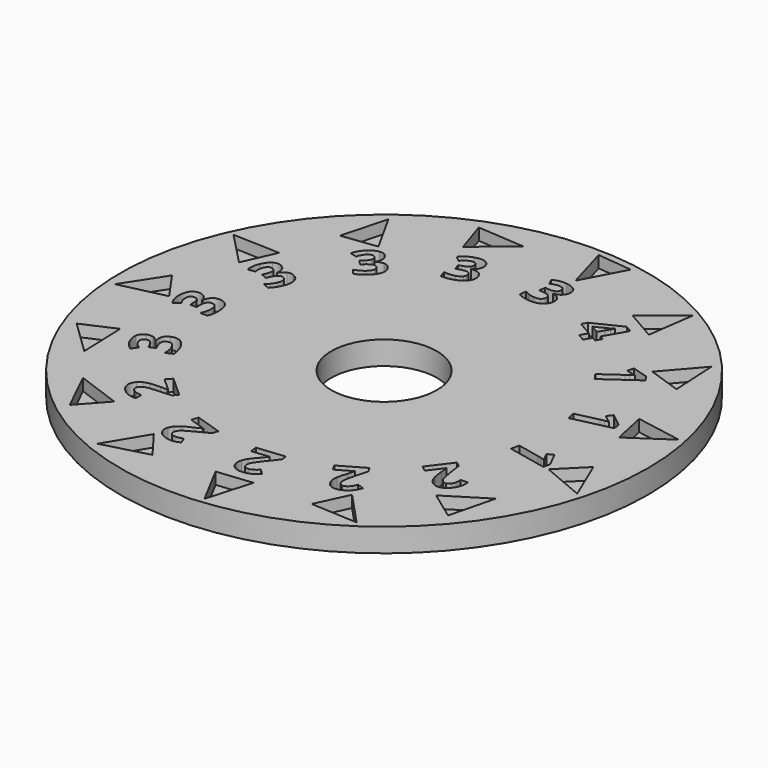
from build123d import *

# Parameters (mm, degrees)
F1_R           = 22.5
F1_R_2         = 4.5
F2_DEPTH       = 2
F1_TEXT_SIZE   = 4.7496985644
F1_TEXT_SIZE_2 = 4.7488933279
F3_DEPTH       = 1


# Not quite as in the source:
# - Text() gives the source's letters only with a copy of the font that has no kerning and outlines rounded to 1/6400 em; it was checked with that copy


with BuildPart() as f2:
    # F1 (on Top) → F2 (new body)
    with BuildSketch(Plane.XY):
        Circle(F1_R)
        Polygon((-11.2424762449, -14.7004235416), (-13.249868064, -16.929858018), (-15.0018269196, -13.3339380845), align=None, mode=Mode.SUBTRACT)
        Polygon((-6.25651676, -16.7168305622), (-4.4510716905, -19.1127370923), (-8.3152139559, -20.1463736594), align=None, mode=Mode.SUBTRACT)
        with BuildLine():
            Line((-10.6299594554, -10.1070689959), (-10.2262327152, -9.6586850257))
            Line((-10.2262327152, -9.6586850257), (-8.4646848666, -11.2447898327))
            Line((-8.4646848666, -11.2447898327), (-8.7983925781, -11.6154097934))
            Line((-8.7983925781, -11.6154097934), (-10.0065299775, -11.6850315037))
            add(Edge.make_bspline(
                [(-10.0065299775, -11.6850315037), (-10.5470234377, -11.7196634778), (-10.7331228689, -11.7533264526)],
                knots=[0, 0, 0, 1, 1, 1], degree=2))
            add(Edge.make_bspline(
                [(-10.7331228689, -11.7533264526), (-10.9192223, -11.7869894275), (-11.0426903114, -11.8475858577)],
                knots=[0, 0, 0, 1, 1, 1], degree=2))
            add(Edge.make_bspline(
                [(-11.0426903114, -11.8475858577), (-11.1661583227, -11.908182288), (-11.2575306723, -12.0096615629)],
                knots=[0, 0, 0, 1, 1, 1], degree=2))
            add(Edge.make_bspline(
                [(-11.2575306723, -12.0096615629), (-11.3940926078, -12.1613289575), (-11.3770531036, -12.3109896076)],
                knots=[0, 0, 0, 1, 1, 1], degree=2))
            add(Edge.make_bspline(
                [(-11.3770531036, -12.3109896076), (-11.3600135994, -12.4606502577), (-11.2204795964, -12.5862872383)],
                knots=[0, 0, 0, 1, 1, 1], degree=2))
            add(Edge.make_bspline(
                [(-11.2204795964, -12.5862872383), (-11.0743273797, -12.7178832852), (-10.8758640896, -12.7747453279)],
                knots=[0, 0, 0, 1, 1, 1], degree=2))
            add(Edge.make_bspline(
                [(-10.8758640896, -12.7747453279), (-10.6774007995, -12.8316073705), (-10.4156554656, -12.8425880348)],
                knots=[0, 0, 0, 1, 1, 1], degree=2))
            Line((-10.4156554656, -12.8425880348), (-10.43498689, -13.446341255))
            add(Edge.make_bspline(
                [(-10.43498689, -13.446341255), (-10.7638659788, -13.4378279364), (-10.9451487095, -13.3929400695)],
                knots=[0, 0, 0, 1, 1, 1], degree=2))
            add(Edge.make_bspline(
                [(-10.9451487095, -13.3929400695), (-11.1264314403, -13.3480522025), (-11.3029865492, -13.2529947668)],
                knots=[0, 0, 0, 1, 1, 1], degree=2))
            add(Edge.make_bspline(
                [(-11.3029865492, -13.2529947668), (-11.4795416581, -13.1579373311), (-11.6587849426, -12.9965459528)],
                knots=[0, 0, 0, 1, 1, 1], degree=2))
            add(Edge.make_bspline(
                [(-11.6587849426, -12.9965459528), (-11.8948345604, -12.7840059223), (-11.9982645368, -12.5350880009)],
                knots=[0, 0, 0, 1, 1, 1], degree=2))
            add(Edge.make_bspline(
                [(-11.9982645368, -12.5350880009), (-12.1016945131, -12.2861700794), (-12.0620052305, -12.0407869417)],
                knots=[0, 0, 0, 1, 1, 1], degree=2))
            add(Edge.make_bspline(
                [(-12.0620052305, -12.0407869417), (-12.0223159479, -11.795403804), (-11.8425507819, -11.5957543609)],
                knots=[0, 0, 0, 1, 1, 1], degree=2))
            add(Edge.make_bspline(
                [(-11.8425507819, -11.5957543609), (-11.6856287033, -11.4214747366), (-11.4871034089, -11.3241014284)],
                knots=[0, 0, 0, 1, 1, 1], degree=2))
            add(Edge.make_bspline(
                [(-11.4871034089, -11.3241014284), (-11.2885781145, -11.2267281201), (-11.0158154046, -11.1822174032)],
                knots=[0, 0, 0, 1, 1, 1], degree=2))
            add(Edge.make_bspline(
                [(-11.0158154046, -11.1822174032), (-10.7430526948, -11.1377066862), (-10.1521469424, -11.1324877692)],
                knots=[0, 0, 0, 1, 1, 1], degree=2))
            Line((-10.1521469424, -11.1324877692), (-9.5532408393, -11.1194926742))
            Line((-9.5532408393, -11.1194926742), (-9.5318875185, -11.0957774088))
            Line((-9.5318875185, -11.0957774088), (-10.6299594554, -10.1070689959))
        make_face(mode=Mode.SUBTRACT)
        with BuildLine():
            Line((-5.6002424488, -13.5567744278), (-5.41379391, -12.9829448295))
            Line((-5.41379391, -12.9829448295), (-3.1594129297, -13.7154376128))
            Line((-3.1594129297, -13.7154376128), (-3.313525375, -14.1897469487))
            Line((-3.313525375, -14.1897469487), (-4.3888961077, -14.7447432961))
            add(Edge.make_bspline(
                [(-4.3888961077, -14.7447432961), (-4.8685753604, -14.9962196744), (-5.0248936849, -15.10266579)],
                knots=[0, 0, 0, 1, 1, 1], degree=2))
            add(Edge.make_bspline(
                [(-5.0248936849, -15.10266579), (-5.1812120095, -15.2091119056), (-5.2693588619, -15.3146884637)],
                knots=[0, 0, 0, 1, 1, 1], degree=2))
            add(Edge.make_bspline(
                [(-5.2693588619, -15.3146884637), (-5.3575057142, -15.4202650218), (-5.3997031695, -15.5501354352)],
                knots=[0, 0, 0, 1, 1, 1], degree=2))
            add(Edge.make_bspline(
                [(-5.3997031695, -15.5501354352), (-5.4627700184, -15.7442352378), (-5.3863311863, -15.8740264542)],
                knots=[0, 0, 0, 1, 1, 1], degree=2))
            add(Edge.make_bspline(
                [(-5.3863311863, -15.8740264542), (-5.3098923542, -16.0038176705), (-5.1313205358, -16.0618391715)],
                knots=[0, 0, 0, 1, 1, 1], degree=2))
            add(Edge.make_bspline(
                [(-5.1313205358, -16.0618391715), (-4.9442789078, -16.1226126804), (-4.7398457943, -16.0938364488)],
                knots=[0, 0, 0, 1, 1, 1], degree=2))
            add(Edge.make_bspline(
                [(-4.7398457943, -16.0938364488), (-4.5354126808, -16.0650602172), (-4.2918301814, -15.9686301347)],
                knots=[0, 0, 0, 1, 1, 1], degree=2))
            Line((-4.2918301814, -15.9686301347), (-4.0639217583, -16.5280489453))
            add(Edge.make_bspline(
                [(-4.0639217583, -16.5280489453), (-4.3678304346, -16.6540388183), (-4.5516979901, -16.6867660406)],
                knots=[0, 0, 0, 1, 1, 1], degree=2))
            add(Edge.make_bspline(
                [(-4.5516979901, -16.6867660406), (-4.7355655457, -16.719493263), (-4.9355200058, -16.7044654068)],
                knots=[0, 0, 0, 1, 1, 1], degree=2))
            add(Edge.make_bspline(
                [(-4.9355200058, -16.7044654068), (-5.1354744658, -16.6894375505), (-5.3648651416, -16.6149040018)],
                knots=[0, 0, 0, 1, 1, 1], degree=2))
            add(Edge.make_bspline(
                [(-5.3648651416, -16.6149040018), (-5.6669550163, -16.5167490515), (-5.8626870411, -16.3314199764)],
                knots=[0, 0, 0, 1, 1, 1], degree=2))
            add(Edge.make_bspline(
                [(-5.8626870411, -16.3314199764), (-6.058419066, -16.1460909013), (-6.1219674158, -15.9057791649)],
                knots=[0, 0, 0, 1, 1, 1], degree=2))
            add(Edge.make_bspline(
                [(-6.1219674158, -15.9057791649), (-6.1855157657, -15.6654674285), (-6.1024968591, -15.4099615065)],
                knots=[0, 0, 0, 1, 1, 1], degree=2))
            add(Edge.make_bspline(
                [(-6.1024968591, -15.4099615065), (-6.0300273163, -15.1869231878), (-5.8882707279, -15.0172207326)],
                knots=[0, 0, 0, 1, 1, 1], degree=2))
            add(Edge.make_bspline(
                [(-5.8882707279, -15.0172207326), (-5.7465141395, -14.8475182773), (-5.5154371445, -14.6959131251)],
                knots=[0, 0, 0, 1, 1, 1], degree=2))
            add(Edge.make_bspline(
                [(-5.5154371445, -14.6959131251), (-5.2843601496, -14.5443079728), (-4.7466636083, -14.2991972328)],
                knots=[0, 0, 0, 1, 1, 1], degree=2))
            Line((-4.7466636083, -14.2991972328), (-4.2048212396, -14.0437285648))
            Line((-4.2048212396, -14.0437285648), (-4.1949598778, -14.0133784139))
            Line((-4.1949598778, -14.0133784139), (-5.6002424488, -13.5567744278))
        make_face(mode=Mode.SUBTRACT)
        Polygon((-20.2206789231, -7.4874351718), (-17.4800425502, -6.2672252426), (-17.3421408981, -10.2648474276), align=None, mode=Mode.SUBTRACT)
        with BuildLine():
            add(Edge.make_bspline(
                [(-16.0555084734, -6.3502361216), (-15.9846522039, -5.9848032435), (-15.63752696, -5.8302531275)],
                knots=[0, 0, 0, 1, 1, 1], degree=2))
            add(Edge.make_bspline(
                [(-15.63752696, -5.8302531275), (-15.3473519515, -5.7010588899), (-15.0656267009, -5.7864377298)],
                knots=[0, 0, 0, 1, 1, 1], degree=2))
            add(Edge.make_bspline(
                [(-15.0656267009, -5.7864377298), (-14.7839014504, -5.8718165696), (-14.5657195033, -6.1556790233)],
                knots=[0, 0, 0, 1, 1, 1], degree=2))
            Line((-14.5657195033, -6.1556790233), (-14.5535158814, -6.1502456208))
            add(Edge.make_bspline(
                [(-14.5535158814, -6.1502456208), (-14.6739633861, -5.7538172162), (-14.5783310232, -5.480524784)],
                knots=[0, 0, 0, 1, 1, 1], degree=2))
            add(Edge.make_bspline(
                [(-14.5783310232, -5.480524784), (-14.4826986603, -5.2072323518), (-14.175574177, -5.0704917219)],
                knots=[0, 0, 0, 1, 1, 1], degree=2))
            add(Edge.make_bspline(
                [(-14.175574177, -5.0704917219), (-13.7287860212, -4.8715688187), (-13.3353417194, -5.0847108089)],
                knots=[0, 0, 0, 1, 1, 1], degree=2))
            add(Edge.make_bspline(
                [(-13.3353417194, -5.0847108089), (-12.9418974175, -5.297852799), (-12.6741514158, -5.8992201649)],
                knots=[0, 0, 0, 1, 1, 1], degree=2))
            add(Edge.make_bspline(
                [(-12.6741514158, -5.8992201649), (-12.4495707785, -6.4036365349), (-12.4434645647, -6.8680328121)],
                knots=[0, 0, 0, 1, 1, 1], degree=2))
            Line((-12.4434645647, -6.8680328121), (-13.0007632961, -7.1161581936))
            add(Edge.make_bspline(
                [(-13.0007632961, -7.1161581936), (-12.9899058705, -6.8960450975), (-13.0289086124, -6.6542629928)],
                knots=[0, 0, 0, 1, 1, 1], degree=2))
            add(Edge.make_bspline(
                [(-13.0289086124, -6.6542629928), (-13.0679113544, -6.4124808881), (-13.1620903313, -6.2009514426)],
                knots=[0, 0, 0, 1, 1, 1], degree=2))
            add(Edge.make_bspline(
                [(-13.1620903313, -6.2009514426), (-13.3066792093, -5.8761995055), (-13.4856738941, -5.7706718458)],
                knots=[0, 0, 0, 1, 1, 1], degree=2))
            add(Edge.make_bspline(
                [(-13.4856738941, -5.7706718458), (-13.6646685788, -5.6651441861), (-13.9087410159, -5.7738122364)],
                knots=[0, 0, 0, 1, 1, 1], degree=2))
            add(Edge.make_bspline(
                [(-13.9087410159, -5.7738122364), (-14.1263722723, -5.8707079146), (-14.1383233267, -6.089276991)],
                knots=[0, 0, 0, 1, 1, 1], degree=2))
            add(Edge.make_bspline(
                [(-14.1383233267, -6.089276991), (-14.1502743812, -6.3078460674), (-13.9767073564, -6.6976839878)],
                knots=[0, 0, 0, 1, 1, 1], degree=2))
            Line((-13.9767073564, -6.6976839878), (-13.8719634301, -6.932942698))
            Line((-13.8719634301, -6.932942698), (-14.3743458632, -7.1566177682))
            Line((-14.3743458632, -7.1566177682), (-14.4809009236, -6.917291184))
            add(Edge.make_bspline(
                [(-14.4809009236, -6.917291184), (-14.6411862978, -6.5572843393), (-14.8095309509, -6.4327984384)],
                knots=[0, 0, 0, 1, 1, 1], degree=2))
            add(Edge.make_bspline(
                [(-14.8095309509, -6.4327984384), (-14.9778756039, -6.3083125375), (-15.2063545242, -6.4100379068)],
                knots=[0, 0, 0, 1, 1, 1], degree=2))
            add(Edge.make_bspline(
                [(-15.2063545242, -6.4100379068), (-15.5582256211, -6.5667010126), (-15.3620194192, -7.0073873574)],
                knots=[0, 0, 0, 1, 1, 1], degree=2))
            add(Edge.make_bspline(
                [(-15.3620194192, -7.0073873574), (-15.2941018877, -7.1599326306), (-15.1729210863, -7.2952625586)],
                knots=[0, 0, 0, 1, 1, 1], degree=2))
            add(Edge.make_bspline(
                [(-15.1729210863, -7.2952625586), (-15.0517402849, -7.4305924866), (-14.8412651329, -7.5675970724)],
                knots=[0, 0, 0, 1, 1, 1], degree=2))
            Line((-14.8412651329, -7.5675970724), (-15.1571916668, -8.0713877192))
            add(Edge.make_bspline(
                [(-15.1571916668, -8.0713877192), (-15.6509420228, -7.7834859121), (-15.9123490549, -7.196356105)],
                knots=[0, 0, 0, 1, 1, 1], degree=2))
            add(Edge.make_bspline(
                [(-15.9123490549, -7.196356105), (-16.1263647428, -6.7156689997), (-16.0555084734, -6.3502361216)],
                knots=[0, 0, 0, 1, 1, 1], degree=2))
        make_face(mode=Mode.SUBTRACT)
        Polygon((0.3273238917, -18.3647082401), (3.3108895778, -18.0511228503), (2.2067086503, -21.8957014331), align=None, mode=Mode.SUBTRACT)
        with BuildLine():
            Line((0.3347819501, -14.5979841554), (0.2717243335, -13.9980310095))
            Line((0.2717243335, -13.9980310095), (2.6287358317, -13.7502991185))
            Line((2.6287358317, -13.7502991185), (2.6808572565, -14.2462013498))
            Line((2.6808572565, -14.2462013498), (1.9243228399, -15.1904483146))
            add(Edge.make_bspline(
                [(1.9243228399, -15.1904483146), (1.5884556461, -15.615214522), (1.4889641565, -15.7760110129)],
                knots=[0, 0, 0, 1, 1, 1], degree=2))
            add(Edge.make_bspline(
                [(1.4889641565, -15.7760110129), (1.389472667, -15.9368075037), (1.3518947371, -16.069086614)],
                knots=[0, 0, 0, 1, 1, 1], degree=2))
            add(Edge.make_bspline(
                [(1.3518947371, -16.069086614), (1.3143168072, -16.2013657243), (1.3285881497, -16.3371484781)],
                knots=[0, 0, 0, 1, 1, 1], degree=2))
            add(Edge.make_bspline(
                [(1.3285881497, -16.3371484781), (1.3499176018, -16.540084659), (1.4725180047, -16.6275495304)],
                knots=[0, 0, 0, 1, 1, 1], degree=2))
            add(Edge.make_bspline(
                [(1.4725180047, -16.6275495304), (1.5951184077, -16.7150144017), (1.7818196942, -16.6953913058)],
                knots=[0, 0, 0, 1, 1, 1], degree=2))
            add(Edge.make_bspline(
                [(1.7818196942, -16.6953913058), (1.9773763777, -16.6748374701), (2.1524012943, -16.5654171897)],
                knots=[0, 0, 0, 1, 1, 1], degree=2))
            add(Edge.make_bspline(
                [(2.1524012943, -16.5654171897), (2.327426211, -16.4559969094), (2.5106971728, -16.2688614487)],
                knots=[0, 0, 0, 1, 1, 1], degree=2))
            Line((2.5106971728, -16.2688614487), (2.9463641336, -16.6871463294))
            add(Edge.make_bspline(
                [(2.9463641336, -16.6871463294), (2.7200128217, -16.9258141311), (2.5653790322, -17.0304798614)],
                knots=[0, 0, 0, 1, 1, 1], degree=2))
            add(Edge.make_bspline(
                [(2.5653790322, -17.0304798614), (2.4107452428, -17.1351455916), (2.2219973789, -17.2027343071)],
                knots=[0, 0, 0, 1, 1, 1], degree=2))
            add(Edge.make_bspline(
                [(2.2219973789, -17.2027343071), (2.033249515, -17.2703230226), (1.7934158466, -17.2955305569)],
                knots=[0, 0, 0, 1, 1, 1], degree=2))
            add(Edge.make_bspline(
                [(1.7934158466, -17.2955305569), (1.477573354, -17.3287269405), (1.2234262199, -17.2390469989)],
                knots=[0, 0, 0, 1, 1, 1], degree=2))
            add(Edge.make_bspline(
                [(1.2234262199, -17.2390469989), (0.9692790858, -17.1493670573), (0.8135076036, -16.9557116414)],
                knots=[0, 0, 0, 1, 1, 1], degree=2))
            add(Edge.make_bspline(
                [(0.8135076036, -16.9557116414), (0.6577361213, -16.7620562255), (0.6296588062, -16.4949184163)],
                knots=[0, 0, 0, 1, 1, 1], degree=2))
            add(Edge.make_bspline(
                [(0.6296588062, -16.4949184163), (0.6051493267, -16.2617262957), (0.6656159542, -16.0490738476)],
                knots=[0, 0, 0, 1, 1, 1], degree=2))
            add(Edge.make_bspline(
                [(0.6656159542, -16.0490738476), (0.7260825818, -15.8364213995), (0.8754932157, -15.6039751344)],
                knots=[0, 0, 0, 1, 1, 1], degree=2))
            add(Edge.make_bspline(
                [(0.8754932157, -15.6039751344), (1.0249038496, -15.3715288692), (1.4163521878, -14.9289832193)],
                knots=[0, 0, 0, 1, 1, 1], degree=2))
            Line((1.4163521878, -14.9289832193), (1.807375051, -14.4752907614))
            Line((1.807375051, -14.4752907614), (1.8040399003, -14.4435589222))
            Line((1.8040399003, -14.4435589222), (0.3347819501, -14.5979841554))
        make_face(mode=Mode.SUBTRACT)
        Polygon((8.2439705729, -18.0201064795), (9.5118253582, -15.3011831184), (12.2385771851, -18.2277552556), align=None, mode=Mode.SUBTRACT)
        with BuildLine():
            Line((6.2546528897, -13.267149647), (5.9529728168, -12.7446244331))
            Line((5.9529728168, -12.7446244331), (8.0057963507, -11.5594262132))
            Line((8.0057963507, -11.5594262132), (8.2551555254, -11.991328973))
            Line((8.2551555254, -11.991328973), (7.9480347187, -13.161850211))
            add(Edge.make_bspline(
                [(7.9480347187, -13.161850211), (7.8139500188, -13.6865919069), (7.7884575235, -13.8739854149)],
                knots=[0, 0, 0, 1, 1, 1], degree=2))
            add(Edge.make_bspline(
                [(7.7884575235, -13.8739854149), (7.7629650282, -14.0613789228), (7.7824419443, -14.1975293063)],
                knots=[0, 0, 0, 1, 1, 1], degree=2))
            add(Edge.make_bspline(
                [(7.7824419443, -14.1975293063), (7.8019188604, -14.3336796899), (7.8701957772, -14.4519387789)],
                knots=[0, 0, 0, 1, 1, 1], degree=2))
            add(Edge.make_bspline(
                [(7.8701957772, -14.4519387789), (7.9722400823, -14.6286846999), (8.1198413152, -14.6587268527)],
                knots=[0, 0, 0, 1, 1, 1], degree=2))
            add(Edge.make_bspline(
                [(8.1198413152, -14.6587268527), (8.267442548, -14.6887690054), (8.4300487954, -14.5948882447)],
                knots=[0, 0, 0, 1, 1, 1], degree=2))
            add(Edge.make_bspline(
                [(8.4300487954, -14.5948882447), (8.600367592, -14.4965546416), (8.7157751376, -14.3253761739)],
                knots=[0, 0, 0, 1, 1, 1], degree=2))
            add(Edge.make_bspline(
                [(8.7157751376, -14.3253761739), (8.8311826832, -14.1541977061), (8.9225096719, -13.9086563125)],
                knots=[0, 0, 0, 1, 1, 1], degree=2))
            Line((8.9225096719, -13.9086563125), (9.4907393676, -14.1136115951))
            add(Edge.make_bspline(
                [(9.4907393676, -14.1136115951), (9.3810134929, -14.4237634354), (9.28230315, -14.5823024441)],
                knots=[0, 0, 0, 1, 1, 1], degree=2))
            add(Edge.make_bspline(
                [(9.28230315, -14.5823024441), (9.183592807, -14.7408414527), (9.0386292843, -14.8793809765)],
                knots=[0, 0, 0, 1, 1, 1], degree=2))
            add(Edge.make_bspline(
                [(9.0386292843, -14.8793809765), (8.8936657615, -15.0179205002), (8.6847842185, -15.1385183153)],
                knots=[0, 0, 0, 1, 1, 1], degree=2))
            add(Edge.make_bspline(
                [(8.6847842185, -15.1385183153), (8.4097032941, -15.2973363611), (8.1410066625, -15.3187842461)],
                knots=[0, 0, 0, 1, 1, 1], degree=2))
            add(Edge.make_bspline(
                [(8.1410066625, -15.3187842461), (7.8723100308, -15.3402321312), (7.6512014615, -15.2266578206)],
                knots=[0, 0, 0, 1, 1, 1], degree=2))
            add(Edge.make_bspline(
                [(7.6512014615, -15.2266578206), (7.4300928923, -15.1130835101), (7.2957654797, -14.8804216067)],
                knots=[0, 0, 0, 1, 1, 1], degree=2))
            add(Edge.make_bspline(
                [(7.2957654797, -14.8804216067), (7.1785072964, -14.6773244756), (7.1472474669, -14.4584256937)],
                knots=[0, 0, 0, 1, 1, 1], degree=2))
            add(Edge.make_bspline(
                [(7.1472474669, -14.4584256937), (7.1159876373, -14.2395269118), (7.1579437427, -13.9663595912)],
                knots=[0, 0, 0, 1, 1, 1], degree=2))
            add(Edge.make_bspline(
                [(7.1579437427, -13.9663595912), (7.1998998481, -13.6931922707), (7.3775362827, -13.1295947702)],
                knots=[0, 0, 0, 1, 1, 1], degree=2))
            Line((7.3775362827, -13.1295947702), (7.5502493767, -12.555985513))
            Line((7.5502493767, -12.555985513), (7.5342933581, -12.5283488781))
            Line((7.5342933581, -12.5283488781), (6.2546528897, -13.267149647))
        make_face(mode=Mode.SUBTRACT)
        Polygon((16.3666587323, -13.6451385915), (13.9396077492, -11.8817828347), (17.3326992901, -9.7635454082), align=None, mode=Mode.SUBTRACT)
        with BuildLine():
            Line((11.116832017, -9.5706739377), (10.6349671793, -9.2075627376))
            Line((10.6349671793, -9.2075627376), (12.0615073676, -7.3144799679))
            Line((12.0615073676, -7.3144799679), (12.4598015508, -7.6146161628))
            Line((12.4598015508, -7.6146161628), (12.6344544419, -8.8120883028))
            add(Edge.make_bspline(
                [(12.6344544419, -8.8120883028), (12.7160617399, -9.3475066468), (12.765816251, -9.5299639919)],
                knots=[0, 0, 0, 1, 1, 1], degree=2))
            add(Edge.make_bspline(
                [(12.765816251, -9.5299639919), (12.8155707622, -9.7124213369), (12.886697551, -9.8301381883)],
                knots=[0, 0, 0, 1, 1, 1], degree=2))
            add(Edge.make_bspline(
                [(12.886697551, -9.8301381883), (12.9578243398, -9.9478550398), (13.0668810805, -10.0300351884)],
                knots=[0, 0, 0, 1, 1, 1], degree=2))
            add(Edge.make_bspline(
                [(13.0668810805, -10.0300351884), (13.2298734918, -10.15285878), (13.3774795472, -10.1228403312)],
                knots=[0, 0, 0, 1, 1, 1], degree=2))
            add(Edge.make_bspline(
                [(13.3774795472, -10.1228403312), (13.5250856027, -10.0928218823), (13.638083307, -9.9428688639)],
                knots=[0, 0, 0, 1, 1, 1], degree=2))
            add(Edge.make_bspline(
                [(13.638083307, -9.9428688639), (13.7564405863, -9.7858034494), (13.7957890362, -9.5831395185)],
                knots=[0, 0, 0, 1, 1, 1], degree=2))
            add(Edge.make_bspline(
                [(13.7957890362, -9.5831395185), (13.8351374862, -9.3804755875), (13.8232637567, -9.1187692457)],
                knots=[0, 0, 0, 1, 1, 1], degree=2))
            Line((13.8232637567, -9.1187692457), (14.4264043583, -9.0854065479))
            add(Edge.make_bspline(
                [(14.4264043583, -9.0854065479), (14.4465871367, -9.413776137), (14.4176699127, -9.5982812676)],
                knots=[0, 0, 0, 1, 1, 1], degree=2))
            add(Edge.make_bspline(
                [(14.4176699127, -9.5982812676), (14.3887526886, -9.7827863982), (14.3094447669, -9.966954463)],
                knots=[0, 0, 0, 1, 1, 1], degree=2))
            add(Edge.make_bspline(
                [(14.3094447669, -9.966954463), (14.2301368451, -10.1511225279), (14.0849816913, -10.3437499231)],
                knots=[0, 0, 0, 1, 1, 1], degree=2))
            add(Edge.make_bspline(
                [(14.0849816913, -10.3437499231), (13.8938235195, -10.597425385), (13.6548673223, -10.7221564054)],
                knots=[0, 0, 0, 1, 1, 1], degree=2))
            add(Edge.make_bspline(
                [(13.6548673223, -10.7221564054), (13.4159111251, -10.8468874258), (13.1680025955, -10.8287357225)],
                knots=[0, 0, 0, 1, 1, 1], degree=2))
            add(Edge.make_bspline(
                [(13.1680025955, -10.8287357225), (12.9200940658, -10.8105840192), (12.7055367825, -10.6489035094)],
                knots=[0, 0, 0, 1, 1, 1], degree=2))
            add(Edge.make_bspline(
                [(12.7055367825, -10.6489035094), (12.5182436845, -10.5077680368), (12.4039382916, -10.3184848341)],
                knots=[0, 0, 0, 1, 1, 1], degree=2))
            add(Edge.make_bspline(
                [(12.4039382916, -10.3184848341), (12.2896328987, -10.1292016314), (12.2215187218, -9.8613562306)],
                knots=[0, 0, 0, 1, 1, 1], degree=2))
            add(Edge.make_bspline(
                [(12.2215187218, -9.8613562306), (12.153404545, -9.5935108298), (12.0967046579, -9.0053085108)],
                knots=[0, 0, 0, 1, 1, 1], degree=2))
            Line((12.0967046579, -9.0053085108), (12.0315609068, -8.4098140234))
            Line((12.0315609068, -8.4098140234), (12.0060748207, -8.3906088799))
            Line((12.0060748207, -8.3906088799), (11.116832017, -9.5706739377))
        make_face(mode=Mode.SUBTRACT)
        with BuildLine():
            Line((16.9413094263, -4.2150202164), (13.624567914, -3.5100250446))
            Line((13.624567914, -3.5100250446), (13.7736213909, -2.8087835692))
            Line((13.7736213909, -2.8087835692), (15.6929614125, -3.2167518849))
            Line((15.6929614125, -3.2167518849), (16.0064689337, -3.2909771683))
            Line((16.0064689337, -3.2909771683), (16.3489677936, -3.3751583522))
            add(Edge.make_bspline(
                [(16.3489677936, -3.3751583522), (16.2117782288, -3.1639049479), (16.1718381834, -3.0840957249)],
                knots=[0, 0, 0, 1, 1, 1], degree=2))
            Line((16.1718381834, -3.0840957249), (15.9465060641, -2.6378717685))
            Line((15.9465060641, -2.6378717685), (16.4401708855, -2.389239825))
            Line((16.4401708855, -2.389239825), (17.0638233608, -3.6386374717))
            Line((17.0638233608, -3.6386374717), (16.9413094263, -4.2150202164))
        make_face(mode=Mode.SUBTRACT)
        Polygon((19.5569883799, -2.1431731293), (21.1183503285, -5.8258554215), (17.4356680363, -4.2644934729), align=None, mode=Mode.SUBTRACT)
        Polygon((-19.5996797298, 1.9013942954), (-17.8789504208, -0.5560618374), (-21.7768121511, -1.4542121207), align=None, mode=Mode.SUBTRACT)
        with BuildLine():
            add(Edge.make_bspline(
                [(-17.2332806051, 0.7788857365), (-17.0199152399, 1.0839054412), (-16.6399393547, 1.0839054412)],
                knots=[0, 0, 0, 1, 1, 1], degree=2))
            add(Edge.make_bspline(
                [(-16.6399393547, 1.0839054412), (-16.3223032632, 1.0839054412), (-16.099661143, 0.8913200072)],
                knots=[0, 0, 0, 1, 1, 1], degree=2))
            add(Edge.make_bspline(
                [(-16.099661143, 0.8913200072), (-15.8770190228, 0.6987345732), (-15.7931571575, 0.3506707253)],
                knots=[0, 0, 0, 1, 1, 1], degree=2))
            Line((-15.7931571575, 0.3506707253), (-15.7797986303, 0.3506707253))
            add(Edge.make_bspline(
                [(-15.7797986303, 0.3506707253), (-15.7285909427, 0.7618165073), (-15.5300683855, 0.9725843811)],
                knots=[0, 0, 0, 1, 1, 1], degree=2))
            add(Edge.make_bspline(
                [(-15.5300683855, 0.9725843811), (-15.3315458283, 1.1833522549), (-14.9953562268, 1.1833522549)],
                knots=[0, 0, 0, 1, 1, 1], degree=2))
            add(Edge.make_bspline(
                [(-14.9953562268, 1.1833522549), (-14.5062857027, 1.1833522549), (-14.2335491055, 0.8286091434)],
                knots=[0, 0, 0, 1, 1, 1], degree=2))
            add(Edge.make_bspline(
                [(-14.2335491055, 0.8286091434), (-13.9608125082, 0.4738660318), (-13.9608125082, -0.1844125036)],
                knots=[0, 0, 0, 1, 1, 1], degree=2))
            add(Edge.make_bspline(
                [(-13.9608125082, -0.1844125036), (-13.9608125082, -0.7365649617), (-14.1441211872, -1.1632956921)],
                knots=[0, 0, 0, 1, 1, 1], degree=2))
            Line((-14.1441211872, -1.1632956921), (-14.7541605966, -1.1632956921))
            add(Edge.make_bspline(
                [(-14.7541605966, -1.1632956921), (-14.6547137829, -0.9666284859), (-14.592002919, -0.7298856981)],
                knots=[0, 0, 0, 1, 1, 1], degree=2))
            add(Edge.make_bspline(
                [(-14.592002919, -0.7298856981), (-14.5292920552, -0.4931429103), (-14.5292920552, -0.2615951053)],
                knots=[0, 0, 0, 1, 1, 1], degree=2))
            add(Edge.make_bspline(
                [(-14.5292920552, -0.2615951053), (-14.5292920552, 0.0938901467), (-14.6498898703, 0.263098158)],
                knots=[0, 0, 0, 1, 1, 1], degree=2))
            add(Edge.make_bspline(
                [(-14.6498898703, 0.263098158), (-14.7704876854, 0.4323061694), (-15.0376582296, 0.4323061694)],
                knots=[0, 0, 0, 1, 1, 1], degree=2))
            add(Edge.make_bspline(
                [(-15.0376582296, 0.4323061694), (-15.2758852983, 0.4323061694), (-15.3757031822, 0.2374943142)],
                knots=[0, 0, 0, 1, 1, 1], degree=2))
            add(Edge.make_bspline(
                [(-15.3757031822, 0.2374943142), (-15.475521066, 0.042682459), (-15.475521066, -0.3840482714)],
                knots=[0, 0, 0, 1, 1, 1], degree=2))
            Line((-15.475521066, -0.3840482714), (-15.475521066, -0.6415709904))
            Line((-15.475521066, -0.6415709904), (-16.025447103, -0.6415709904))
            Line((-16.025447103, -0.6415709904), (-16.025447103, -0.379595429))
            add(Edge.make_bspline(
                [(-16.025447103, -0.379595429), (-16.025447103, 0.0144811238), (-16.1286046187, 0.1966765922)],
                knots=[0, 0, 0, 1, 1, 1], degree=2))
            add(Edge.make_bspline(
                [(-16.1286046187, 0.1966765922), (-16.2317621344, 0.3788720605), (-16.4818634494, 0.3788720605)],
                knots=[0, 0, 0, 1, 1, 1], degree=2))
            add(Edge.make_bspline(
                [(-16.4818634494, 0.3788720605), (-16.8670343173, 0.3788720605), (-16.8670343173, -0.1035191999)],
                knots=[0, 0, 0, 1, 1, 1], degree=2))
            add(Edge.make_bspline(
                [(-16.8670343173, -0.1035191999), (-16.8670343173, -0.2705007901), (-16.8113737873, -0.4434195034)],
                knots=[0, 0, 0, 1, 1, 1], degree=2))
            add(Edge.make_bspline(
                [(-16.8113737873, -0.4434195034), (-16.7557132572, -0.6163382168), (-16.6191594235, -0.8271060906)],
                knots=[0, 0, 0, 1, 1, 1], degree=2))
            Line((-16.6191594235, -0.8271060906), (-17.11268279, -1.1588428497))
            add(Edge.make_bspline(
                [(-17.11268279, -1.1588428497), (-17.4466459703, -0.6950050993), (-17.4466459703, -0.0523115123)],
                knots=[0, 0, 0, 1, 1, 1], degree=2))
            add(Edge.make_bspline(
                [(-17.4466459703, -0.0523115123), (-17.4466459703, 0.4738660318), (-17.2332806051, 0.7788857365)],
                knots=[0, 0, 0, 1, 1, 1], degree=2))
        make_face(mode=Mode.SUBTRACT)
        Polygon((-16.0679658148, 8.8988833145), (-17.2881757441, 6.1582469416), (-20.0655879999, 9.0367849666), align=None, mode=Mode.SUBTRACT)
        with BuildLine():
            add(Edge.make_bspline(
                [(-15.5222102597, 7.5285174245), (-15.2032286088, 7.7203832778), (-14.8561033649, 7.5658331618)],
                knots=[0, 0, 0, 1, 1, 1], degree=2))
            add(Edge.make_bspline(
                [(-14.8561033649, 7.5658331618), (-14.5659283563, 7.4366389243), (-14.4408662116, 7.1701466673)],
                knots=[0, 0, 0, 1, 1, 1], degree=2))
            add(Edge.make_bspline(
                [(-14.4408662116, 7.1701466673), (-14.315804067, 6.9036544103), (-14.380762762, 6.5515725695)],
                knots=[0, 0, 0, 1, 1, 1], degree=2))
            Line((-14.380762762, 6.5515725695), (-14.3685591401, 6.5461391669))
            add(Edge.make_bspline(
                [(-14.3685591401, 6.5461391669), (-14.1545505345, 6.9009114855), (-13.8874641367, 7.0127111208)],
                knots=[0, 0, 0, 1, 1, 1], degree=2))
            add(Edge.make_bspline(
                [(-13.8874641367, 7.0127111208), (-13.6203777389, 7.124510756), (-13.3132532555, 6.987770126)],
                knots=[0, 0, 0, 1, 1, 1], degree=2))
            add(Edge.make_bspline(
                [(-13.3132532555, 6.987770126), (-12.8664650998, 6.7888472229), (-12.7615948426, 6.3538412967)],
                knots=[0, 0, 0, 1, 1, 1], degree=2))
            add(Edge.make_bspline(
                [(-12.7615948426, 6.3538412967), (-12.6567245853, 5.9188353705), (-12.924470587, 5.3174680046)],
                knots=[0, 0, 0, 1, 1, 1], degree=2))
            add(Edge.make_bspline(
                [(-12.924470587, 5.3174680046), (-13.1490512243, 4.8130516346), (-13.4900790601, 4.4977720709)],
                knots=[0, 0, 0, 1, 1, 1], degree=2))
            Line((-13.4900790601, 4.4977720709), (-14.0473777915, 4.7458974524))
            add(Edge.make_bspline(
                [(-14.0473777915, 4.7458974524), (-13.8765368474, 4.8851132221), (-13.7229556557, 5.0758817143)],
                knots=[0, 0, 0, 1, 1, 1], degree=2))
            add(Edge.make_bspline(
                [(-13.7229556557, 5.0758817143), (-13.5693744641, 5.2666502065), (-13.4751954872, 5.478179652)],
                knots=[0, 0, 0, 1, 1, 1], degree=2))
            add(Edge.make_bspline(
                [(-13.4751954872, 5.478179652), (-13.3306066092, 5.8029315892), (-13.3719550969, 6.0065623498)],
                knots=[0, 0, 0, 1, 1, 1], degree=2))
            add(Edge.make_bspline(
                [(-13.3719550969, 6.0065623498), (-13.4133035845, 6.2101931105), (-13.6573760216, 6.3188611608)],
                knots=[0, 0, 0, 1, 1, 1], degree=2))
            add(Edge.make_bspline(
                [(-13.6573760216, 6.3188611608), (-13.8750072781, 6.415756839), (-14.0454325725, 6.2783869446)],
                knots=[0, 0, 0, 1, 1, 1], degree=2))
            add(Edge.make_bspline(
                [(-14.0454325725, 6.2783869446), (-14.2158578669, 6.1410170502), (-14.3894248917, 5.7511791298)],
                knots=[0, 0, 0, 1, 1, 1], degree=2))
            Line((-14.3894248917, 5.7511791298), (-14.494168818, 5.5159204196))
            Line((-14.494168818, 5.5159204196), (-14.996551251, 5.7395954898))
            Line((-14.996551251, 5.7395954898), (-14.8899961906, 5.978922074))
            add(Edge.make_bspline(
                [(-14.8899961906, 5.978922074), (-14.7297108164, 6.3389289187), (-14.7498443231, 6.5473307029)],
                knots=[0, 0, 0, 1, 1, 1], degree=2))
            add(Edge.make_bspline(
                [(-14.7498443231, 6.5473307029), (-14.7699778298, 6.7557324871), (-14.9984567501, 6.8574578564)],
                knots=[0, 0, 0, 1, 1, 1], degree=2))
            add(Edge.make_bspline(
                [(-14.9984567501, 6.8574578564), (-15.3503278469, 7.0141209622), (-15.5465340489, 6.5734346174)],
                knots=[0, 0, 0, 1, 1, 1], degree=2))
            add(Edge.make_bspline(
                [(-15.5465340489, 6.5734346174), (-15.6144515803, 6.4208893442), (-15.6339355329, 6.2402810619)],
                knots=[0, 0, 0, 1, 1, 1], degree=2))
            add(Edge.make_bspline(
                [(-15.6339355329, 6.2402810619), (-15.6534194855, 6.0596727797), (-15.6143983684, 5.811585298)],
                knots=[0, 0, 0, 1, 1, 1], degree=2))
            Line((-15.6143983684, 5.811585298), (-16.2001838939, 5.7092627259))
            add(Edge.make_bspline(
                [(-16.2001838939, 5.7092627259), (-16.3166146307, 6.2688346588), (-16.0552075986, 6.8559644659)],
                knots=[0, 0, 0, 1, 1, 1], degree=2))
            add(Edge.make_bspline(
                [(-16.0552075986, 6.8559644659), (-15.8411919107, 7.3366515712), (-15.5222102597, 7.5285174245)],
                knots=[0, 0, 0, 1, 1, 1], degree=2))
        make_face(mode=Mode.SUBTRACT)
        Polygon((-11.4671495317, 13.7284078013), (-14.4447879866, 13.3627997711), (-13.4078723792, 17.2260634203), align=None, mode=Mode.SUBTRACT)
        with BuildLine():
            add(Edge.make_bspline(
                [(-10.9438926203, 13.2139988204), (-10.5744495089, 13.2595354732), (-10.3201960145, 12.9771583604)],
                knots=[0, 0, 0, 1, 1, 1], degree=2))
            add(Edge.make_bspline(
                [(-10.3201960145, 12.9771583604), (-10.107655984, 12.7411087426), (-10.1017981958, 12.4467885948)],
                knots=[0, 0, 0, 1, 1, 1], degree=2))
            add(Edge.make_bspline(
                [(-10.1017981958, 12.4467885948), (-10.0959404076, 12.152468447), (-10.2984877144, 11.8572467622)],
                knots=[0, 0, 0, 1, 1, 1], degree=2))
            Line((-10.2984877144, 11.8572467622), (-10.289549115, 11.8473194418))
            add(Edge.make_bspline(
                [(-10.289549115, 11.8473194418), (-9.9497436235, 12.0843749401), (-9.6602750497, 12.0778751642)],
                knots=[0, 0, 0, 1, 1, 1], degree=2))
            add(Edge.make_bspline(
                [(-9.6602750497, 12.0778751642), (-9.3708064758, 12.0713753883), (-9.1458517239, 11.8215378255)],
                knots=[0, 0, 0, 1, 1, 1], degree=2))
            add(Edge.make_bspline(
                [(-9.1458517239, 11.8215378255), (-8.8185996676, 11.4580875963), (-8.8997287706, 11.018035332)],
                knots=[0, 0, 0, 1, 1, 1], degree=2))
            add(Edge.make_bspline(
                [(-8.8997287706, 11.018035332), (-8.9808578736, 10.5779830677), (-9.4700541609, 10.1375087522)],
                knots=[0, 0, 0, 1, 1, 1], degree=2))
            add(Edge.make_bspline(
                [(-9.4700541609, 10.1375087522), (-9.880383403, 9.7680466431), (-10.3201635847, 9.6187329469)],
                knots=[0, 0, 0, 1, 1, 1], degree=2))
            Line((-10.3201635847, 9.6187329469), (-10.7283596246, 10.0720805773))
            add(Edge.make_bspline(
                [(-10.7283596246, 10.0720805773), (-10.5156645012, 10.1297732392), (-10.2977685651, 10.2415818304)],
                knots=[0, 0, 0, 1, 1, 1], degree=2))
            add(Edge.make_bspline(
                [(-10.2977685651, 10.2415818304), (-10.079872629, 10.3533904216), (-9.9077990759, 10.5083261448)],
                knots=[0, 0, 0, 1, 1, 1], degree=2))
            add(Edge.make_bspline(
                [(-9.9077990759, 10.5083261448), (-9.6436220504, 10.746192207), (-9.5985716815, 10.9490361085)],
                knots=[0, 0, 0, 1, 1, 1], degree=2))
            add(Edge.make_bspline(
                [(-9.5985716815, 10.9490361085), (-9.5535213126, 11.15188001), (-9.7322933008, 11.3504264175)],
                knots=[0, 0, 0, 1, 1, 1], degree=2))
            add(Edge.make_bspline(
                [(-9.7322933008, 11.3504264175), (-9.8916983237, 11.5274636308), (-10.103262947, 11.4712881999)],
                knots=[0, 0, 0, 1, 1, 1], degree=2))
            add(Edge.make_bspline(
                [(-10.103262947, 11.4712881999), (-10.3148275703, 11.415112769), (-10.6319503045, 11.1295741766)],
                knots=[0, 0, 0, 1, 1, 1], degree=2))
            Line((-10.6319503045, 11.1295741766), (-10.8233269806, 10.9572578435))
            Line((-10.8233269806, 10.9572578435), (-11.1912993231, 11.3659325322))
            Line((-11.1912993231, 11.3659325322), (-10.9966135402, 11.5412283985))
            add(Edge.make_bspline(
                [(-10.9966135402, 11.5412283985), (-10.7037575892, 11.8049170812), (-10.6373858207, 12.0034906194)],
                knots=[0, 0, 0, 1, 1, 1], degree=2))
            add(Edge.make_bspline(
                [(-10.6373858207, 12.0034906194), (-10.5710140521, 12.2020641577), (-10.7383644967, 12.3879256558)],
                knots=[0, 0, 0, 1, 1, 1], degree=2))
            add(Edge.make_bspline(
                [(-10.7383644967, 12.3879256558), (-10.9960941131, 12.6741633932), (-11.3545806822, 12.3513806366)],
                knots=[0, 0, 0, 1, 1, 1], degree=2))
            add(Edge.make_bspline(
                [(-11.3545806822, 12.3513806366), (-11.4786721869, 12.2396481439), (-11.5699316697, 12.0825791055)],
                knots=[0, 0, 0, 1, 1, 1], degree=2))
            add(Edge.make_bspline(
                [(-11.5699316697, 12.0825791055), (-11.6611911526, 11.9255100671), (-11.7264498578, 11.682999557)],
                knots=[0, 0, 0, 1, 1, 1], degree=2))
            Line((-11.7264498578, 11.682999557), (-12.3032099032, 11.8277836743))
            add(Edge.make_bspline(
                [(-12.3032099032, 11.8277836743), (-12.1819762644, 12.3863347188), (-11.7043618509, 12.8163806684)],
                knots=[0, 0, 0, 1, 1, 1], degree=2))
            add(Edge.make_bspline(
                [(-11.7043618509, 12.8163806684), (-11.3133357317, 13.1684621675), (-10.9438926203, 13.2139988204)],
                knots=[0, 0, 0, 1, 1, 1], degree=2))
        make_face(mode=Mode.SUBTRACT)
        with BuildLine():
            add(Edge.make_bspline(
                [(-4.6724472064, 16.5377611259), (-4.3164227048, 16.4290948773), (-4.1990036988, 16.0677163357)],
                knots=[0, 0, 0, 1, 1, 1], degree=2))
            add(Edge.make_bspline(
                [(-4.1990036988, 16.0677163357), (-4.1008487485, 15.7656264611), (-4.2152081817, 15.4943690499)],
                knots=[0, 0, 0, 1, 1, 1], degree=2))
            add(Edge.make_bspline(
                [(-4.2152081817, 15.4943690499), (-4.3295676148, 15.2231116387), (-4.6346812639, 15.0357966211)],
                knots=[0, 0, 0, 1, 1, 1], degree=2))
            Line((-4.6346812639, 15.0357966211), (-4.630553252, 15.0230919068))
            add(Edge.make_bspline(
                [(-4.630553252, 15.0230919068), (-4.2237063311, 15.1014415356), (-3.9619073274, 14.9777662188)],
                knots=[0, 0, 0, 1, 1, 1], degree=2))
            add(Edge.make_bspline(
                [(-3.9619073274, 14.9777662188), (-3.7001083237, 14.854090902), (-3.5962200235, 14.5343555908)],
                knots=[0, 0, 0, 1, 1, 1], degree=2))
            add(Edge.make_bspline(
                [(-3.5962200235, 14.5343555908), (-3.4450889201, 14.069221882), (-3.6981894244, 13.7002123138)],
                knots=[0, 0, 0, 1, 1, 1], degree=2))
            add(Edge.make_bspline(
                [(-3.6981894244, 13.7002123138), (-3.9512899287, 13.3312027457), (-4.5773500193, 13.1277834912)],
                knots=[0, 0, 0, 1, 1, 1], degree=2))
            add(Edge.make_bspline(
                [(-4.5773500193, 13.1277834912), (-5.1024782126, 12.9571589981), (-5.5649687514, 12.9996288641)],
                knots=[0, 0, 0, 1, 1, 1], degree=2))
            Line((-5.5649687514, 12.9996288641), (-5.7534812962, 13.5798108195))
            add(Edge.make_bspline(
                [(-5.7534812962, 13.5798108195), (-5.5357089127, 13.5460047883), (-5.291174419, 13.5595207573)],
                knots=[0, 0, 0, 1, 1, 1], degree=2))
            add(Edge.make_bspline(
                [(-5.291174419, 13.5595207573), (-5.0466399253, 13.5730367263), (-4.8264248765, 13.6445889331)],
                knots=[0, 0, 0, 1, 1, 1], degree=2))
            add(Edge.make_bspline(
                [(-4.8264248765, 13.6445889331), (-4.4883383112, 13.7544399172), (-4.3646787038, 13.9214234062)],
                knots=[0, 0, 0, 1, 1, 1], degree=2))
            add(Edge.make_bspline(
                [(-4.3646787038, 13.9214234062), (-4.2410190963, 14.0884068952), (-4.3235793349, 14.3425011823)],
                knots=[0, 0, 0, 1, 1, 1], degree=2))
            add(Edge.make_bspline(
                [(-4.3235793349, 14.3425011823), (-4.3971955476, 14.5690685882), (-4.6133180544, 14.6038008632)],
                knots=[0, 0, 0, 1, 1, 1], degree=2))
            add(Edge.make_bspline(
                [(-4.6133180544, 14.6038008632), (-4.8294405612, 14.6385331382), (-5.235285603, 14.5066660905)],
                knots=[0, 0, 0, 1, 1, 1], degree=2))
            Line((-5.235285603, 14.5066660905), (-5.4802042631, 14.4270871938))
            Line((-5.4802042631, 14.4270871938), (-5.6501407541, 14.9500979347))
            Line((-5.6501407541, 14.9500979347), (-5.4009871893, 15.0310528353))
            add(Edge.make_bspline(
                [(-5.4009871893, 15.0310528353), (-5.0261981159, 15.1528291872), (-4.8847973539, 15.3072393107)],
                knots=[0, 0, 0, 1, 1, 1], degree=2))
            add(Edge.make_bspline(
                [(-4.8847973539, 15.3072393107), (-4.7433965919, 15.4616494343), (-4.8206821486, 15.6995099197)],
                knots=[0, 0, 0, 1, 1, 1], degree=2))
            add(Edge.make_bspline(
                [(-4.8206821486, 15.6995099197), (-4.9397064925, 16.0658291835), (-5.3984878442, 15.9167620861)],
                knots=[0, 0, 0, 1, 1, 1], degree=2))
            add(Edge.make_bspline(
                [(-5.3984878442, 15.9167620861), (-5.5572967736, 15.865161937), (-5.704552193, 15.7587908061)],
                knots=[0, 0, 0, 1, 1, 1], degree=2))
            add(Edge.make_bspline(
                [(-5.704552193, 15.7587908061), (-5.8518076124, 15.6524196752), (-6.010062317, 15.457418407)],
                knots=[0, 0, 0, 1, 1, 1], degree=2))
            Line((-6.010062317, 15.457418407), (-6.4780698308, 15.8242747244))
            add(Edge.make_bspline(
                [(-6.4780698308, 15.8242747244), (-6.1401342139, 16.2852263307), (-5.52889629, 16.4838295713)],
                knots=[0, 0, 0, 1, 1, 1], degree=2))
            add(Edge.make_bspline(
                [(-5.52889629, 16.4838295713), (-5.028471708, 16.6464273745), (-4.6724472064, 16.5377611259)],
                knots=[0, 0, 0, 1, 1, 1], degree=2))
        make_face(mode=Mode.SUBTRACT)
        Polygon((-7.043811027, 17.2027386725), (-7.9708620101, 20.0559082214), (-3.9807245699, 19.77518913), align=None, mode=Mode.SUBTRACT)
        Circle(F1_R_2, mode=Mode.SUBTRACT)
        with BuildLine():
            Line((17.1770722576, 3.0935315605), (13.8731397634, 2.330758642))
            Line((13.8731397634, 2.330758642), (13.7118706368, 3.029291973))
            Line((13.7118706368, 3.029291973), (15.6237983047, 3.4706952553))
            Line((15.6237983047, 3.4706952553), (15.9393015728, 3.5359183066))
            Line((15.9393015728, 3.5359183066), (16.2852874622, 3.6043705169))
            add(Edge.make_bspline(
                [(16.2852874622, 3.6043705169), (16.0716719447, 3.7378523069), (16.0017451355, 3.7933046346)],
                knots=[0, 0, 0, 1, 1, 1], degree=2))
            Line((16.0017451355, 3.7933046346), (15.6089424884, 4.1024914125))
            Line((15.6089424884, 4.1024914125), (15.9512783603, 4.5364602477))
            Line((15.9512783603, 4.5364602477), (17.0445177167, 3.6676883564))
            Line((17.0445177167, 3.6676883564), (17.1770722576, 3.0935315605))
        make_face(mode=Mode.SUBTRACT)
        Polygon((18.2298897834, 2.2451655079), (17.6061547109, 5.1796083101), (21.5450906255, 4.4833440924), align=None, mode=Mode.SUBTRACT)
        with BuildLine():
            Line((14.4709389179, 9.7723817203), (11.7032078745, 7.8134388105))
            Line((11.7032078745, 7.8134388105), (11.2890387236, 8.3986058466))
            Line((11.2890387236, 8.3986058466), (12.8906760356, 9.5322116801))
            Line((12.8906760356, 9.5322116801), (13.1578646331, 9.7122300457))
            Line((13.1578646331, 9.7122300457), (13.4520332453, 9.9067982043))
            add(Edge.make_bspline(
                [(13.4520332453, 9.9067982043), (13.2037509628, 9.9492821509), (13.1180165654, 9.9740678808)],
                knots=[0, 0, 0, 1, 1, 1], degree=2))
            Line((13.1180165654, 9.9740678808), (12.6372926591, 10.1111624069))
            Line((12.6372926591, 10.1111624069), (12.7894450645, 10.6425496901))
            Line((12.7894450645, 10.6425496901), (14.1305141707, 10.2533575242))
            Line((14.1305141707, 10.2533575242), (14.4709389179, 9.7723817203))
        make_face(mode=Mode.SUBTRACT)
        with BuildLine():
            add(Edge.make_bspline(
                [(2.4386634821, 17.0902087368), (2.7197095032, 16.8461289684), (2.6799912079, 16.4682346309)],
                knots=[0, 0, 0, 1, 1, 1], degree=2))
            add(Edge.make_bspline(
                [(2.6799912079, 16.4682346309), (2.6467891954, 16.1523385831), (2.4319863259, 15.9510467792)],
                knots=[0, 0, 0, 1, 1, 1], degree=2))
            add(Edge.make_bspline(
                [(2.4319863259, 15.9510467792), (2.2171834563, 15.7497549753), (1.8622603867, 15.7027350932)],
                knots=[0, 0, 0, 1, 1, 1], degree=2))
            Line((1.8622603867, 15.7027350932), (1.8608640404, 15.6894497454))
            add(Edge.make_bspline(
                [(1.8608640404, 15.6894497454), (2.2644048618, 15.5955461421), (2.4532668694, 15.3760798703)],
                knots=[0, 0, 0, 1, 1, 1], degree=2))
            add(Edge.make_bspline(
                [(2.4532668694, 15.3760798703), (2.6421288769, 15.1566135985), (2.6069874944, 14.8222656788)],
                knots=[0, 0, 0, 1, 1, 1], degree=2))
            add(Edge.make_bspline(
                [(2.6069874944, 14.8222656788), (2.5558657041, 14.3358743342), (2.1745571751, 14.1017125689)],
                knots=[0, 0, 0, 1, 1, 1], degree=2))
            add(Edge.make_bspline(
                [(2.1745571751, 14.1017125689), (1.7932486461, 13.8675508036), (1.1385762293, 13.9363596473)],
                knots=[0, 0, 0, 1, 1, 1], degree=2))
            add(Edge.make_bspline(
                [(1.1385762293, 13.9363596473), (0.5894485202, 13.9940752952), (0.1842164399, 14.2209852975)],
                knots=[0, 0, 0, 1, 1, 1], degree=2))
            Line((0.1842164399, 14.2209852975), (0.2479829219, 14.8276828472))
            add(Edge.make_bspline(
                [(0.2479829219, 14.8276828472), (0.4331777419, 14.7082234927), (0.6620685577, 14.6211098057)],
                knots=[0, 0, 0, 1, 1, 1], degree=2))
            add(Edge.make_bspline(
                [(0.6620685577, 14.6211098057), (0.8909593736, 14.5339961187), (1.1212387355, 14.5097927825)],
                knots=[0, 0, 0, 1, 1, 1], degree=2))
            add(Edge.make_bspline(
                [(1.1212387355, 14.5097927825), (1.474776602, 14.4726344554), (1.6556635785, 14.5748845697)],
                knots=[0, 0, 0, 1, 1, 1], degree=2))
            add(Edge.make_bspline(
                [(1.6556635785, 14.5748845697), (1.8365505549, 14.6771346839), (1.8644774813, 14.94284164)],
                knots=[0, 0, 0, 1, 1, 1], degree=2))
            add(Edge.make_bspline(
                [(1.8644774813, 14.94284164), (1.8893789907, 15.1797636758), (1.7060681453, 15.2993981307)],
                knots=[0, 0, 0, 1, 1, 1], degree=2))
            add(Edge.make_bspline(
                [(1.7060681453, 15.2993981307), (1.5227572998, 15.4190325857), (1.098364245, 15.4636380931)],
                knots=[0, 0, 0, 1, 1, 1], degree=2))
            Line((1.098364245, 15.4636380931), (0.8422522624, 15.4905565472))
            Line((0.8422522624, 15.4905565472), (0.8997351859, 16.0374700318))
            Line((0.8997351859, 16.0374700318), (1.1602756178, 16.0100861289))
            add(Edge.make_bspline(
                [(1.1602756178, 16.0100861289), (1.552193378, 15.9688939124), (1.7441736571, 16.0524417081)],
                knots=[0, 0, 0, 1, 1, 1], degree=2))
            add(Edge.make_bspline(
                [(1.7441736571, 16.0524417081), (1.9361539363, 16.1359895039), (1.9622966424, 16.3847207377)],
                knots=[0, 0, 0, 1, 1, 1], degree=2))
            add(Edge.make_bspline(
                [(1.9622966424, 16.3847207377), (2.0025579613, 16.7677815994), (1.5228092907, 16.8182052165)],
                knots=[0, 0, 0, 1, 1, 1], degree=2))
            add(Edge.make_bspline(
                [(1.5228092907, 16.8182052165), (1.3567424431, 16.8356595455), (1.1789528869, 16.7983788571)],
                knots=[0, 0, 0, 1, 1, 1], degree=2))
            add(Edge.make_bspline(
                [(1.1789528869, 16.7983788571), (1.0011633307, 16.7610981686), (0.7772763029, 16.647323633)],
                knots=[0, 0, 0, 1, 1, 1], degree=2))
            Line((0.7772763029, 16.647323633), (0.4989440716, 17.1728193605))
            add(Edge.make_bspline(
                [(0.4989440716, 17.1728193605), (0.9951495283, 17.4564688083), (1.6343223726, 17.3892890353)],
                knots=[0, 0, 0, 1, 1, 1], degree=2))
            add(Edge.make_bspline(
                [(1.6343223726, 17.3892890353), (2.1576174611, 17.3342885052), (2.4386634821, 17.0902087368)],
                knots=[0, 0, 0, 1, 1, 1], degree=2))
        make_face(mode=Mode.SUBTRACT)
        Polygon((8.5233473456, 12.6490317448), (8.2450446954, 12.1669974147), (7.8915528533, 12.3710860249), (7.5401493736, 11.762437344), (6.93342883, 12.1127276131), (7.2848323098, 12.721376294), (6.0315430514, 13.4449631847), (6.2809022261, 13.8768659445), (8.6635550472, 15.0292429615), (9.2355691189, 14.6989904832), (8.1698555036, 12.853120355), align=None, mode=Mode.SUBTRACT)
        Polygon((0.73933148, 21.9412472285), (3.7228971661, 21.6276618387), (1.8435124075, 18.0966686457), align=None, mode=Mode.SUBTRACT)
        Polygon((7.9316178638, 16.5497572192), (11.0847055912, 19.0110653639), (10.5296940751, 15.0497572192), align=None, mode=Mode.SUBTRACT)
        Polygon((16.8712437153, 10.0646940991), (14.0346879885, 11.0413985625), (16.6602048792, 14.0591230458), align=None, mode=Mode.SUBTRACT)
    extrude(amount=F2_DEPTH)



with BuildPart() as f2b:
    # F1 (on Top) → F2, piece 2 (new body)
    with BuildSketch(Plane.XY):
        with BuildLine():
            Line((6.8561512758, 13.6115878445), (7.56313496, 13.2034106241))
            Line((7.56313496, 13.2034106241), (7.8507143653, 13.7015127652))
            add(Edge.make_bspline(
                [(7.8507143653, 13.7015127652), (7.9227019842, 13.8261989786), (8.069724752, 14.0571013896)],
                knots=[0, 0, 0, 1, 1, 1], degree=2))
            add(Edge.make_bspline(
                [(8.069724752, 14.0571013896), (8.2167475199, 14.2880038006), (8.2447961439, 14.3232269152)],
                knots=[0, 0, 0, 1, 1, 1], degree=2))
            Line((8.2447961439, 14.3232269152), (8.2287283329, 14.3325036703))
            add(Edge.make_bspline(
                [(8.2287283329, 14.3325036703), (8.0588086483, 14.2103707164), (7.8645191743, 14.1143049659)],
                knots=[0, 0, 0, 1, 1, 1], degree=2))
            Line((7.8645191743, 14.1143049659), (6.8561512758, 13.6115878445))
        make_face()
    extrude(amount=F2_DEPTH)


with BuildPart() as f2_1:
    add(f2.part)

    add(f2b.part)  # F3 merges F2b
    # F1 (on Top) → F3 (join)
    with BuildSketch(Plane.XY):
        Polygon((17.4356680363, -4.2644934729), (21.1183503285, -5.8258554215), (19.5569883799, -2.1431731293), align=None)
        Polygon((21.5450906255, 4.4833440924), (17.6061547109, 5.1796083101), (18.2298897834, 2.2451655079), align=None)
        Polygon((17.3326992901, -9.7635454082), (13.9396077492, -11.8817828347), (16.3666587323, -13.6451385915), align=None)
        with Locations(Location((12.1758449656, -7.1627488505), (0, 0, -127))):
            Text('2', F1_TEXT_SIZE, font='Open Sans', font_style=FontStyle.BOLD, text_align=(TextAlign.LEFT, TextAlign.BOTTOM))
        with Locations(Location((8.1703307354, -11.4644322419), (0, 0, -150))):
            Text('2', F1_TEXT_SIZE, font='Open Sans', font_style=FontStyle.BOLD, text_align=(TextAlign.LEFT, TextAlign.BOTTOM))
        with Locations(Location((2.8176509675, -13.7304433376), (0, 0, -174))):
            Text('2', F1_TEXT_SIZE_2, font='Open Sans', font_style=FontStyle.BOLD, text_align=(TextAlign.LEFT, TextAlign.BOTTOM))
        with Locations(Location((-2.9787236589, -13.7741471158), (0, 0, 162))):
            Text('2', F1_TEXT_SIZE, font='Open Sans', font_style=FontStyle.BOLD, text_align=(TextAlign.LEFT, TextAlign.BOTTOM))
        Polygon((-15.0018269196, -13.3339380845), (-13.249868064, -16.929858018), (-11.2424762449, -14.7004235416), align=None)
        Polygon((-17.3421408981, -10.2648474276), (-17.4800425502, -6.2672252426), (-20.2206789231, -7.4874351718), align=None)
        Polygon((-8.3152139559, -20.1463736594), (-4.4510716905, -19.1127370923), (-6.25651676, -16.7168305622), align=None)
        Polygon((2.2067086503, -21.8957014331), (3.3108895778, -18.0511228503), (0.3273238917, -18.3647082401), align=None)
        Polygon((12.2385771851, -18.2277552556), (9.5118253582, -15.3011831184), (8.2439705729, -18.0201064795), align=None)
        Polygon((16.6602048792, 14.0591230458), (14.0346879885, 11.0413985625), (16.8712437153, 10.0646940991), align=None)
        Polygon((10.5296940751, 15.0497572192), (11.0847055912, 19.0110653639), (7.9316178638, 16.5497572192), align=None)
        Polygon((-21.7768121511, -1.4542121207), (-17.8789504208, -0.5560618374), (-19.5996797298, 1.9013942954), align=None)
        Polygon((-20.0655879999, 9.0367849666), (-17.2881757441, 6.1582469416), (-16.0679658148, 8.8988833145), align=None)
        Polygon((-13.4078723792, 17.2260634203), (-14.4447879866, 13.3627997711), (-11.4671495317, 13.7284078013), align=None)
        Polygon((-3.9807245699, 19.77518913), (-7.9708620101, 20.0559082214), (-7.043811027, 17.2027386725), align=None)
        Polygon((1.8435124075, 18.0966686457), (3.7228971661, 21.6276618387), (0.73933148, 21.9412472285), align=None)
        with Locations(Location((-5.6949907574, 12.8138009556), (0, 0, 18))):
            Text('3', F1_TEXT_SIZE, font='Open Sans', font_style=FontStyle.BOLD, text_align=(TextAlign.LEFT, TextAlign.BOTTOM))
        with Locations(Location((-0.0101475927, 14.1041077701), (0, 0, -6))):
            Text('3', F1_TEXT_SIZE, font='Open Sans', font_style=FontStyle.BOLD, text_align=(TextAlign.LEFT, TextAlign.BOTTOM))
        with Locations(Location((5.6100839157, 12.8767611557), (0, 0, -30))):
            Text('4', F1_TEXT_SIZE, font='Open Sans', font_style=FontStyle.BOLD, text_align=(TextAlign.LEFT, TextAlign.BOTTOM))
        with Locations(Location((-10.363361578, 9.396085991), (0, 0, 42))):
            Text('3', F1_TEXT_SIZE, font='Open Sans', font_style=FontStyle.BOLD, text_align=(TextAlign.LEFT, TextAlign.BOTTOM))
        with Locations(Location((-13.4389837152, 4.276803749), (0, 0, 66))):
            Text('3', F1_TEXT_SIZE, font='Open Sans', font_style=FontStyle.BOLD, text_align=(TextAlign.LEFT, TextAlign.BOTTOM))
        with Locations(Location((-14.0075673535, -1.3443779499), (0, 0, 90))):
            Text('3', F1_TEXT_SIZE, font='Open Sans', font_style=FontStyle.BOLD, text_align=(TextAlign.LEFT, TextAlign.BOTTOM))
        with Locations(Location((-12.2450636406, -6.9779182382), (0, 0, 114))):
            Text('3', F1_TEXT_SIZE, font='Open Sans', font_style=FontStyle.BOLD, text_align=(TextAlign.LEFT, TextAlign.BOTTOM))
        with Locations(Location((-8.3234963102, -11.37191658), (0, 0, 138))):
            Text('2', F1_TEXT_SIZE, font='Open Sans', font_style=FontStyle.BOLD, text_align=(TextAlign.LEFT, TextAlign.BOTTOM))
        with Locations(Location((14.0325362296, -1.590685023), (0, 0, -102))):
            Text('1', F1_TEXT_SIZE, font='Open Sans', font_style=FontStyle.BOLD, text_align=(TextAlign.LEFT, TextAlign.BOTTOM))
        with Locations(Location((13.4317364811, 4.2426863099), (0, 0, -77))):
            Text('1', F1_TEXT_SIZE, font='Open Sans', font_style=FontStyle.BOLD, text_align=(TextAlign.LEFT, TextAlign.BOTTOM))
        with Locations(Location((10.5696020411, 9.4150761226), (0, 0, -54.7099277999))):
            Text('1', F1_TEXT_SIZE, font='Open Sans', font_style=FontStyle.BOLD, text_align=(TextAlign.LEFT, TextAlign.BOTTOM))
    extrude(amount=F3_DEPTH)


solid = f2_1.part
